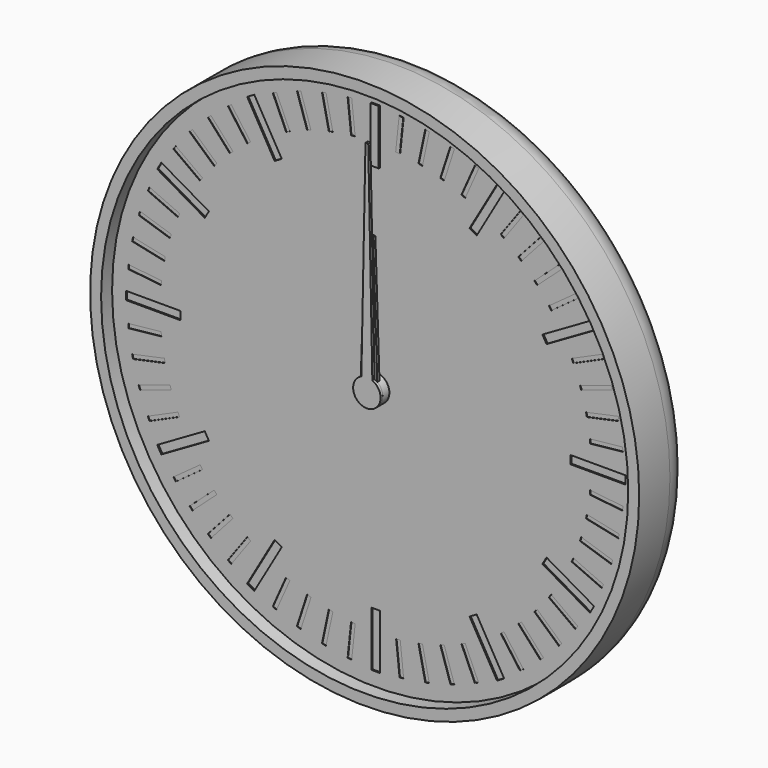
from build123d import *

# Parameters (mm, degrees)
F0_R      = 100
F1_DEPTH  = 24
F2_R      = 10
F3_T      = -4
F4_R      = 5
F4_R_2    = 3
F5_DEPTH  = 2
F6_DEPTH  = 19
F7_DEPTH  = 8
F9_DEPTH  = 4
F11_DEPTH = 4
F12_R     = 5
F12_R_2   = 3
F13_DEPTH = 2
F14_R     = 3
F15_DEPTH = 4
F17_DEPTH = 4
F18_R     = 3
F19_DEPTH = 2
F20_R     = 98
F20_R_2   = 5
F21_DEPTH = 1
F23_R     = 5
F23_R_2   = 3
F24_DEPTH = 2
F25_W     = 3
F25_H     = 20
F25_W_2   = 20
F25_H_2   = 3
F26_DEPTH = 0.5
F27_W     = 1.5
F27_H     = 12
F27_W_2   = 12
F27_H_2   = 1.5
F28_DEPTH = 0.2
F29_DEPTH = 1
F30_DEPTH = 0.4
F31_R     = 5
F31_R_2   = 3
F32_DEPTH = 5
F33_R     = 3
F34_DEPTH = 1
F36_DEPTH = 1


with BuildPart() as f1:
    # F0 (on Front) → F1 (new body)
    with BuildSketch(Plane.XZ):
        Circle(F0_R)
    extrude(amount=F1_DEPTH)

    # F2
    f2_edges = [f1.edges().sort_by_distance(p)[0] for p in [
        (-100, 0, 0),
    ]]
    fillet(f2_edges, radius=F2_R)

    # F3
    f3_openings = [f1.faces().sort_by_distance(p)[0] for p in [
        (0, -24, 0),
    ]]
    offset(amount=F3_T, openings=f3_openings)

    # F4 (on face) → F5 (join)
    with BuildSketch(Plane.XZ.offset(4)):
        Circle(F4_R)
        Circle(F4_R_2, mode=Mode.SUBTRACT)
        with Locations((40, 0)):
            Circle(F4_R)
        with Locations((40, 0)):
            Circle(F4_R_2, mode=Mode.SUBTRACT)
    extrude(amount=F5_DEPTH)


with BuildPart() as f6:
    # F6 (new): a face of the model
    f6_faces = [f1.part.faces().sort_by_distance(p)[0] for p in [
        (0, -4, 0),
    ]]
    extrude(f6_faces, amount=F6_DEPTH)

    # F8 (on face) → F9 (join)
    with BuildSketch(Plane.XZ.offset(6)):
        with BuildLine():
            ThreePointArc((9.2729637667, -1.3794085621), (9.3494561423, -0.6915886375), (9.375, 0))
            ThreePointArc((9.375, 0), (9.3494561423, 0.6915886375), (9.2729637667, 1.3794085621))
            ThreePointArc((9.2729637667, 1.3794085621), (8.9161548403, 2.8970343223), (8.3127812852, 4.3345463782))
            ThreePointArc((8.3127812852, 4.3345463782), (7.5845343223, 5.5104867402), (6.6911892658, 6.566476316))
            ThreePointArc((6.6911892658, 6.566476316), (5.5104867402, 7.5845343223), (4.1773988938, 8.3928519278))
            ThreePointArc((4.1773988938, 8.3928519278), (2.8970343223, 8.9161548403), (1.5536078905, 9.2453733036))
            ThreePointArc((1.5536078905, 9.2453733036), (0, 9.375), (-1.5536078905, 9.2453733036))
            ThreePointArc((-1.5536078905, 9.2453733036), (-2.8970343223, 8.9161548403), (-4.1773988938, 8.3928519278))
            ThreePointArc((-4.1773988938, 8.3928519278), (-5.5104867402, 7.5845343223), (-6.6911892658, 6.566476316))
            ThreePointArc((-6.6911892658, 6.566476316), (-7.5845343223, 5.5104867402), (-8.3127812852, 4.3345463782))
            ThreePointArc((-8.3127812852, 4.3345463782), (-8.9161548403, 2.8970343223), (-9.2729637667, 1.3794085621))
            ThreePointArc((-9.2729637667, 1.3794085621), (-9.375, 0), (-9.2729637667, -1.3794085621))
            ThreePointArc((-9.2729637667, -1.3794085621), (-8.9161548403, -2.8970343223), (-8.3127812852, -4.3345463782))
            ThreePointArc((-8.3127812852, -4.3345463782), (-7.5845343223, -5.5104867402), (-6.6911892658, -6.566476316))
            ThreePointArc((-6.6911892658, -6.566476316), (-5.5104867402, -7.5845343223), (-4.1773988938, -8.3928519278))
            ThreePointArc((-4.1773988938, -8.3928519278), (-2.8970343223, -8.9161548403), (-1.5536078905, -9.2453733036))
            ThreePointArc((-1.5536078905, -9.2453733036), (0, -9.375), (1.5536078905, -9.2453733036))
            ThreePointArc((1.5536078905, -9.2453733036), (2.8970343223, -8.9161548403), (4.1773988938, -8.3928519278))
            ThreePointArc((4.1773988938, -8.3928519278), (5.5104867402, -7.5845343223), (6.6911892658, -6.566476316))
            ThreePointArc((6.6911892658, -6.566476316), (7.5845343223, -5.5104867402), (8.3127812852, -4.3345463782))
            ThreePointArc((8.3127812852, -4.3345463782), (8.9161548403, -2.8970343223), (9.2729637667, -1.3794085621))
        make_face()
        with BuildLine():
            ThreePointArc((8.3127812852, 4.3345463782), (8.9161548403, 2.8970343223), (9.2729637667, 1.3794085621))
            Line((9.2729637667, 1.3794085621), (11.1823199426, 2.3946312492))
            Line((11.1823199426, 2.3946312492), (10.8182678729, 3.515068311))
            Line((10.8182678729, 3.515068311), (10.4542158031, 4.6355053728))
            Line((10.4542158031, 4.6355053728), (8.3127812852, 4.3345463782))
        make_face()
        with BuildLine():
            Line((11.1823199426, -2.3946312492), (9.2729637667, -1.3794085621))
            ThreePointArc((9.2729637667, -1.3794085621), (8.9161548403, -2.8970343223), (8.3127812852, -4.3345463782))
            Line((8.3127812852, -4.3345463782), (10.4542158031, -4.6355053728))
            Line((10.4542158031, -4.6355053728), (10.8182678729, -3.515068311))
            Line((10.8182678729, -3.515068311), (11.1823199426, -2.3946312492))
        make_face()
        with BuildLine():
            ThreePointArc((4.1773988938, 8.3928519278), (5.5104867402, 7.5845343223), (6.6911892658, 6.566476316))
            Line((6.6911892658, 6.566476316), (7.6391579371, 8.5101001246))
            Line((7.6391579371, 8.5101001246), (6.6860572448, 9.202568311))
            Line((6.6860572448, 9.202568311), (5.7329565525, 9.8950364974))
            Line((5.7329565525, 9.8950364974), (4.1773988938, 8.3928519278))
        make_face()
        with BuildLine():
            Line((7.6391579371, -8.5101001246), (6.6911892658, -6.566476316))
            ThreePointArc((6.6911892658, -6.566476316), (5.5104867402, -7.5845343223), (4.1773988938, -8.3928519278))
            Line((4.1773988938, -8.3928519278), (5.7329565525, -9.8950364974))
            Line((5.7329565525, -9.8950364974), (6.6860572448, -9.202568311))
            Line((6.6860572448, -9.202568311), (7.6391579371, -8.5101001246))
        make_face()
        with BuildLine():
            ThreePointArc((-1.5536078905, 9.2453733036), (0, 9.375), (1.5536078905, 9.2453733036))
            Line((1.5536078905, 9.2453733036), (1.1780972451, 11.375))
            Line((1.1780972451, 11.375), (0, 11.375))
            Line((0, 11.375), (-1.1780972451, 11.375))
            Line((-1.1780972451, 11.375), (-1.5536078905, 9.2453733036))
        make_face()
        with BuildLine():
            Line((1.1780972451, -11.375), (1.5536078905, -9.2453733036))
            ThreePointArc((1.5536078905, -9.2453733036), (0, -9.375), (-1.5536078905, -9.2453733036))
            Line((-1.5536078905, -9.2453733036), (-1.1780972451, -11.375))
            Line((-1.1780972451, -11.375), (0, -11.375))
            Line((0, -11.375), (1.1780972451, -11.375))
        make_face()
        with BuildLine():
            ThreePointArc((-6.6911892658, 6.566476316), (-5.5104867402, 7.5845343223), (-4.1773988938, 8.3928519278))
            Line((-4.1773988938, 8.3928519278), (-5.7329565525, 9.8950364974))
            Line((-5.7329565525, 9.8950364974), (-6.6860572448, 9.202568311))
            Line((-6.6860572448, 9.202568311), (-7.6391579371, 8.5101001246))
            Line((-7.6391579371, 8.5101001246), (-6.6911892658, 6.566476316))
        make_face()
        with BuildLine():
            Line((-5.7329565525, -9.8950364974), (-4.1773988938, -8.3928519278))
            ThreePointArc((-4.1773988938, -8.3928519278), (-5.5104867402, -7.5845343223), (-6.6911892658, -6.566476316))
            Line((-6.6911892658, -6.566476316), (-7.6391579371, -8.5101001246))
            Line((-7.6391579371, -8.5101001246), (-6.6860572448, -9.202568311))
            Line((-6.6860572448, -9.202568311), (-5.7329565525, -9.8950364974))
        make_face()
        with BuildLine():
            ThreePointArc((-9.2729637667, 1.3794085621), (-8.9161548403, 2.8970343223), (-8.3127812852, 4.3345463782))
            Line((-8.3127812852, 4.3345463782), (-10.4542158031, 4.6355053728))
            Line((-10.4542158031, 4.6355053728), (-10.8182678729, 3.515068311))
            Line((-10.8182678729, 3.515068311), (-11.1823199426, 2.3946312492))
            Line((-11.1823199426, 2.3946312492), (-9.2729637667, 1.3794085621))
        make_face()
        with BuildLine():
            Line((-10.4542158031, -4.6355053728), (-8.3127812852, -4.3345463782))
            ThreePointArc((-8.3127812852, -4.3345463782), (-8.9161548403, -2.8970343223), (-9.2729637667, -1.3794085621))
            Line((-9.2729637667, -1.3794085621), (-11.1823199426, -2.3946312492))
            Line((-11.1823199426, -2.3946312492), (-10.8182678729, -3.515068311))
            Line((-10.8182678729, -3.515068311), (-10.4542158031, -4.6355053728))
        make_face()
    extrude(amount=F9_DEPTH)

    # F35 (on face) → F36 (join)
    with BuildSketch(Plane.XZ.offset(23)):
        with BuildLine():
            ThreePointArc((-2, 4.582575695), (-2.7386127875, -4.1833001327), (5, 0))
            ThreePointArc((5, 0), (4.1833001327, 2.7386127875), (2, 4.582575695))
            ThreePointArc((2, 4.582575695), (0, 5), (-2, 4.582575695))
        make_face()
        with BuildLine():
            ThreePointArc((-2, 4.582575695), (0, 5), (2, 4.582575695))
            Line((2, 4.582575695), (0.5, 80))
            Line((0.5, 80), (0, 80))
            Line((0, 80), (-0.5, 80))
            Line((-0.5, 80), (-2, 4.582575695))
        make_face()
    extrude(amount=-F36_DEPTH)


with BuildPart() as f7:
    # F7 (new): a face of the model
    f7_faces = [f1.part.faces().sort_by_distance(p)[0] for p in [
        (40, -4, 0),
    ]]
    extrude(f7_faces, amount=F7_DEPTH)

    # F10 (on face) → F11 (join)
    with BuildSketch(Plane.XZ.offset(6)):
        with BuildLine():
            ThreePointArc((68.0833122289, -1.5307512065), (68.1145761255, -0.765659377), (68.125, 0))
            ThreePointArc((68.125, 0), (68.1145761255, 0.765659377), (68.0833122289, 1.5307512065))
            ThreePointArc((68.0833122289, 1.5307512065), (67.9709283072, 2.9398630294), (67.7878855489, 4.3415483093))
            ThreePointArc((67.7878855489, 4.3415483093), (67.5104012706, 5.8475163042), (67.1513634058, 7.3361495492))
            ThreePointArc((67.1513634058, 7.3361495492), (66.7484645208, 8.6911029668), (66.2779949294, 10.0241013309))
            ThreePointArc((66.2779949294, 10.0241013309), (65.6934659962, 11.4394680865), (65.0327697151, 12.8209229539))
            ThreePointArc((65.0327697151, 12.8209229539), (64.3569644814, 14.0625), (63.6196298356, 15.2685530234))
            ThreePointArc((63.6196298356, 15.2685530234), (62.7536029668, 16.5314602207), (61.8201238674, 17.7453605039))
            ThreePointArc((61.8201238674, 17.7453605039), (60.9009482166, 18.8192983038), (59.9289735785, 19.8456956821))
            ThreePointArc((59.9289735785, 19.8456956821), (58.8192983038, 20.9009482166), (57.6538339021, 21.8942406481))
            ThreePointArc((57.6538339021, 21.8942406481), (56.5314602207, 22.7536029668), (55.3673255461, 23.5554862093))
            ThreePointArc((55.3673255461, 23.5554862093), (54.0625, 24.3569644814), (52.7159866827, 25.0862374159))
            ThreePointArc((52.7159866827, 25.0862374159), (51.4394680865, 25.6934659962), (50.1340516468, 26.2357889574))
            ThreePointArc((50.1340516468, 26.2357889574), (48.6911029668, 26.7484645208), (47.2223898273, 27.1818452314))
            ThreePointArc((47.2223898273, 27.1818452314), (45.8475163042, 27.5104012706), (44.457871062, 27.7694618348))
            ThreePointArc((44.457871062, 27.7694618348), (42.9398630294, 27.9709283072), (41.4131398795, 28.0894759773))
            ThreePointArc((41.4131398795, 28.0894759773), (40, 28.125), (38.5868601205, 28.0894759773))
            ThreePointArc((38.5868601205, 28.0894759773), (37.0601369706, 27.9709283072), (35.542128938, 27.7694618348))
            ThreePointArc((35.542128938, 27.7694618348), (34.1524836958, 27.5104012706), (32.7776101727, 27.1818452314))
            ThreePointArc((32.7776101727, 27.1818452314), (31.3088970332, 26.7484645208), (29.8659483532, 26.2357889574))
            ThreePointArc((29.8659483532, 26.2357889574), (28.5605319135, 25.6934659962), (27.2840133173, 25.0862374159))
            ThreePointArc((27.2840133173, 25.0862374159), (25.9375, 24.3569644814), (24.6326744539, 23.5554862093))
            ThreePointArc((24.6326744539, 23.5554862093), (23.4685397793, 22.7536029668), (22.3461660979, 21.8942406481))
            ThreePointArc((22.3461660979, 21.8942406481), (21.1807016962, 20.9009482166), (20.0710264215, 19.8456956821))
            ThreePointArc((20.0710264215, 19.8456956821), (19.0990517834, 18.8192983038), (18.1798761326, 17.7453605039))
            ThreePointArc((18.1798761326, 17.7453605039), (17.2463970332, 16.5314602207), (16.3803701644, 15.2685530234))
            ThreePointArc((16.3803701644, 15.2685530234), (15.6430355186, 14.0625), (14.9672302849, 12.8209229539))
            ThreePointArc((14.9672302849, 12.8209229539), (14.3065340038, 11.4394680865), (13.7220050706, 10.0241013309))
            ThreePointArc((13.7220050706, 10.0241013309), (13.2515354792, 8.6911029668), (12.8486365942, 7.3361495492))
            ThreePointArc((12.8486365942, 7.3361495492), (12.4895987294, 5.8475163042), (12.2121144511, 4.3415483093))
            ThreePointArc((12.2121144511, 4.3415483093), (12.0290716928, 2.9398630294), (11.9166877711, 1.5307512065))
            ThreePointArc((11.9166877711, 1.5307512065), (11.875, 0), (11.9166877711, -1.5307512065))
            ThreePointArc((11.9166877711, -1.5307512065), (12.0290716928, -2.9398630294), (12.2121144511, -4.3415483093))
            ThreePointArc((12.2121144511, -4.3415483093), (12.4895987294, -5.8475163042), (12.8486365942, -7.3361495492))
            ThreePointArc((12.8486365942, -7.3361495492), (13.2515354792, -8.6911029668), (13.7220050706, -10.0241013309))
            ThreePointArc((13.7220050706, -10.0241013309), (14.3065340038, -11.4394680865), (14.9672302849, -12.8209229539))
            ThreePointArc((14.9672302849, -12.8209229539), (15.6430355186, -14.0625), (16.3803701644, -15.2685530234))
            ThreePointArc((16.3803701644, -15.2685530234), (17.2463970332, -16.5314602207), (18.1798761326, -17.7453605039))
            ThreePointArc((18.1798761326, -17.7453605039), (19.0990517834, -18.8192983038), (20.0710264215, -19.8456956821))
            ThreePointArc((20.0710264215, -19.8456956821), (21.1807016962, -20.9009482166), (22.3461660979, -21.8942406481))
            ThreePointArc((22.3461660979, -21.8942406481), (23.4685397793, -22.7536029668), (24.6326744539, -23.5554862093))
            ThreePointArc((24.6326744539, -23.5554862093), (25.9375, -24.3569644814), (27.2840133173, -25.0862374159))
            ThreePointArc((27.2840133173, -25.0862374159), (28.5605319135, -25.6934659962), (29.8659483532, -26.2357889574))
            ThreePointArc((29.8659483532, -26.2357889574), (31.3088970332, -26.7484645208), (32.7776101727, -27.1818452314))
            ThreePointArc((32.7776101727, -27.1818452314), (34.1524836958, -27.5104012706), (35.542128938, -27.7694618348))
            ThreePointArc((35.542128938, -27.7694618348), (37.0601369706, -27.9709283072), (38.5868601205, -28.0894759773))
            ThreePointArc((38.5868601205, -28.0894759773), (40, -28.125), (41.4131398795, -28.0894759773))
            ThreePointArc((41.4131398795, -28.0894759773), (42.9398630294, -27.9709283072), (44.457871062, -27.7694618348))
            ThreePointArc((44.457871062, -27.7694618348), (45.8475163042, -27.5104012706), (47.2223898273, -27.1818452314))
            ThreePointArc((47.2223898273, -27.1818452314), (48.6911029668, -26.7484645208), (50.1340516468, -26.2357889574))
            ThreePointArc((50.1340516468, -26.2357889574), (51.4394680865, -25.6934659962), (52.7159866827, -25.0862374159))
            ThreePointArc((52.7159866827, -25.0862374159), (54.0625, -24.3569644814), (55.3673255461, -23.5554862093))
            ThreePointArc((55.3673255461, -23.5554862093), (56.5314602207, -22.7536029668), (57.6538339021, -21.8942406481))
            ThreePointArc((57.6538339021, -21.8942406481), (58.8192983038, -20.9009482166), (59.9289735785, -19.8456956821))
            ThreePointArc((59.9289735785, -19.8456956821), (60.9009482166, -18.8192983038), (61.8201238674, -17.7453605039))
            ThreePointArc((61.8201238674, -17.7453605039), (62.7536029668, -16.5314602207), (63.6196298356, -15.2685530234))
            ThreePointArc((63.6196298356, -15.2685530234), (64.3569644814, -14.0625), (65.0327697151, -12.8209229539))
            ThreePointArc((65.0327697151, -12.8209229539), (65.6934659962, -11.4394680865), (66.2779949294, -10.0241013309))
            ThreePointArc((66.2779949294, -10.0241013309), (66.7484645208, -8.6911029668), (67.1513634058, -7.3361495492))
            ThreePointArc((67.1513634058, -7.3361495492), (67.5104012706, -5.8475163042), (67.7878855489, -4.3415483093))
            ThreePointArc((67.7878855489, -4.3415483093), (67.9709283072, -2.9398630294), (68.0833122289, -1.5307512065))
        make_face()
        with BuildLine():
            ThreePointArc((68.0833122289, 1.5307512065), (68.1145761255, 0.765659377), (68.125, 0))
            ThreePointArc((68.125, 0), (68.1145761255, -0.765659377), (68.0833122289, -1.5307512065))
            Line((68.0833122289, -1.5307512065), (70.0833122289, -1.1780972451))
            Line((70.0833122289, -1.1780972451), (70.0833122289, 0))
            Line((70.0833122289, 0), (70.0833122289, 1.1780972451))
            Line((70.0833122289, 1.1780972451), (68.0833122289, 1.5307512065))
        make_face()
        with BuildLine():
            ThreePointArc((67.1513634058, 7.3361495492), (67.5104012706, 5.8475163042), (67.7878855489, 4.3415483093))
            Line((67.7878855489, 4.3415483093), (69.670859869, 5.1023193172))
            Line((69.670859869, 5.1023193172), (69.4259196788, 6.2546723109))
            Line((69.4259196788, 6.2546723109), (69.1809794886, 7.4070253046))
            Line((69.1809794886, 7.4070253046), (67.1513634058, 7.3361495492))
        make_face()
        with BuildLine():
            Line((69.670859869, -5.1023193172), (67.7878855489, -4.3415483093))
            ThreePointArc((67.7878855489, -4.3415483093), (67.5104012706, -5.8475163042), (67.1513634058, -7.3361495492))
            Line((67.1513634058, -7.3361495492), (69.1809794886, -7.4070253046))
            Line((69.1809794886, -7.4070253046), (69.4259196788, -6.2546723109))
            Line((69.4259196788, -6.2546723109), (69.670859869, -5.1023193172))
        make_face()
        with BuildLine():
            ThreePointArc((65.0327697151, 12.8209229539), (65.6934659962, 11.4394680865), (66.2779949294, 10.0241013309))
            Line((66.2779949294, 10.0241013309), (67.9616485562, 11.1597400416))
            Line((67.9616485562, 11.1597400416), (67.4824732375, 12.2359854286))
            Line((67.4824732375, 12.2359854286), (67.0032979188, 13.3122308155))
            Line((67.0032979188, 13.3122308155), (65.0327697151, 12.8209229539))
        make_face()
        with BuildLine():
            Line((67.9616485562, -11.1597400416), (66.2779949294, -10.0241013309))
            ThreePointArc((66.2779949294, -10.0241013309), (65.6934659962, -11.4394680865), (65.0327697151, -12.8209229539))
            Line((65.0327697151, -12.8209229539), (67.0032979188, -13.3122308155))
            Line((67.0032979188, -13.3122308155), (67.4824732375, -12.2359854286))
            Line((67.4824732375, -12.2359854286), (67.9616485562, -11.1597400416))
        make_face()
        with BuildLine():
            ThreePointArc((61.8201238674, 17.7453605039), (62.7536029668, 16.5314602207), (63.6196298356, 15.2685530234))
            Line((63.6196298356, 15.2685530234), (65.0303790267, 16.7294265759))
            Line((65.0303790267, 16.7294265759), (64.3379108402, 17.6825272682))
            Line((64.3379108402, 17.6825272682), (63.6454426538, 18.6356279605))
            Line((63.6454426538, 18.6356279605), (61.8201238674, 17.7453605039))
        make_face()
        with BuildLine():
            Line((65.0303790267, -16.7294265759), (63.6196298356, -15.2685530234))
            ThreePointArc((63.6196298356, -15.2685530234), (62.7536029668, -16.5314602207), (61.8201238674, -17.7453605039))
            Line((61.8201238674, -17.7453605039), (63.6454426538, -18.6356279605))
            Line((63.6454426538, -18.6356279605), (64.3379108402, -17.6825272682))
            Line((64.3379108402, -17.6825272682), (65.0303790267, -16.7294265759))
        make_face()
        with BuildLine():
            ThreePointArc((57.6538339021, 21.8942406481), (58.8192983038, 20.9009482166), (59.9289735785, 19.8456956821))
            Line((59.9289735785, 19.8456956821), (61.0051618246, 21.5679568921))
            Line((61.0051618246, 21.5679568921), (60.129664953, 22.3562578161))
            Line((60.129664953, 22.3562578161), (59.2541680814, 23.1445587401))
            Line((59.2541680814, 23.1445587401), (57.6538339021, 21.8942406481))
        make_face()
        with BuildLine():
            Line((61.0051618246, -21.5679568921), (59.9289735785, -19.8456956821))
            ThreePointArc((59.9289735785, -19.8456956821), (58.8192983038, -20.9009482166), (57.6538339021, -21.8942406481))
            Line((57.6538339021, -21.8942406481), (59.2541680814, -23.1445587401))
            Line((59.2541680814, -23.1445587401), (60.129664953, -22.3562578161))
            Line((60.129664953, -22.3562578161), (61.0051618246, -21.5679568921))
        make_face()
        with BuildLine():
            ThreePointArc((52.7159866827, 25.0862374159), (54.0625, 24.3569644814), (55.3673255461, 23.5554862093))
            Line((55.3673255461, 23.5554862093), (56.0619182568, 25.4638639976))
            Line((56.0619182568, 25.4638639976), (55.0416561144, 26.0529126202))
            Line((55.0416561144, 26.0529126202), (54.021393972, 26.6419612427))
            Line((54.021393972, 26.6419612427), (52.7159866827, 25.0862374159))
        make_face()
        with BuildLine():
            Line((56.0619182568, -25.4638639976), (55.3673255461, -23.5554862093))
            ThreePointArc((55.3673255461, -23.5554862093), (54.0625, -24.3569644814), (52.7159866827, -25.0862374159))
            Line((52.7159866827, -25.0862374159), (54.021393972, -26.6419612427))
            Line((54.021393972, -26.6419612427), (55.0416561144, -26.0529126202))
            Line((55.0416561144, -26.0529126202), (56.0619182568, -25.4638639976))
        make_face()
        with BuildLine():
            ThreePointArc((47.2223898273, 27.1818452314), (48.6911029668, 26.7484645208), (50.1340516468, 26.2357889574))
            Line((50.1340516468, 26.2357889574), (50.4166917876, 28.2468780572))
            Line((50.4166917876, 28.2468780572), (49.2962547258, 28.610930127))
            Line((49.2962547258, 28.610930127), (48.175817664, 28.9749821968))
            Line((48.175817664, 28.9749821968), (47.2223898273, 27.1818452314))
        make_face()
        with BuildLine():
            Line((50.4166917876, -28.2468780572), (50.1340516468, -26.2357889574))
            ThreePointArc((50.1340516468, -26.2357889574), (48.6911029668, -26.7484645208), (47.2223898273, -27.1818452314))
            Line((47.2223898273, -27.1818452314), (48.175817664, -28.9749821968))
            Line((48.175817664, -28.9749821968), (49.2962547258, -28.610930127))
            Line((49.2962547258, -28.610930127), (50.4166917876, -28.2468780572))
        make_face()
        with BuildLine():
            ThreePointArc((41.4131398795, 28.0894759773), (42.9398630294, 27.9709283072), (44.457871062, 27.7694618348))
            Line((44.457871062, 27.7694618348), (44.3162059024, 29.7953680022))
            Line((44.3162059024, 29.7953680022), (43.1445623973, 29.9185126968))
            Line((43.1445623973, 29.9185126968), (41.9729188922, 30.0416573914))
            Line((41.9729188922, 30.0416573914), (41.4131398795, 28.0894759773))
        make_face()
        with BuildLine():
            Line((44.3162059024, -29.7953680022), (44.457871062, -27.7694618348))
            ThreePointArc((44.457871062, -27.7694618348), (42.9398630294, -27.9709283072), (41.4131398795, -28.0894759773))
            Line((41.4131398795, -28.0894759773), (41.9729188922, -30.0416573914))
            Line((41.9729188922, -30.0416573914), (43.1445623973, -29.9185126968))
            Line((43.1445623973, -29.9185126968), (44.3162059024, -29.7953680022))
        make_face()
        with BuildLine():
            ThreePointArc((35.542128938, 27.7694618348), (37.0601369706, 27.9709283072), (38.5868601205, 28.0894759773))
            Line((38.5868601205, 28.0894759773), (38.0270811078, 30.0416573914))
            Line((38.0270811078, 30.0416573914), (36.8554376027, 29.9185126968))
            Line((36.8554376027, 29.9185126968), (35.6837940976, 29.7953680022))
            Line((35.6837940976, 29.7953680022), (35.542128938, 27.7694618348))
        make_face()
        with BuildLine():
            Line((38.0270811078, -30.0416573914), (38.5868601205, -28.0894759773))
            ThreePointArc((38.5868601205, -28.0894759773), (37.0601369706, -27.9709283072), (35.542128938, -27.7694618348))
            Line((35.542128938, -27.7694618348), (35.6837940976, -29.7953680022))
            Line((35.6837940976, -29.7953680022), (36.8554376027, -29.9185126968))
            Line((36.8554376027, -29.9185126968), (38.0270811078, -30.0416573914))
        make_face()
        with BuildLine():
            ThreePointArc((29.8659483532, 26.2357889574), (31.3088970332, 26.7484645208), (32.7776101727, 27.1818452314))
            Line((32.7776101727, 27.1818452314), (31.824182336, 28.9749821968))
            Line((31.824182336, 28.9749821968), (30.7037452742, 28.610930127))
            Line((30.7037452742, 28.610930127), (29.5833082124, 28.2468780572))
            Line((29.5833082124, 28.2468780572), (29.8659483532, 26.2357889574))
        make_face()
        with BuildLine():
            Line((31.824182336, -28.9749821968), (32.7776101727, -27.1818452314))
            ThreePointArc((32.7776101727, -27.1818452314), (31.3088970332, -26.7484645208), (29.8659483532, -26.2357889574))
            Line((29.8659483532, -26.2357889574), (29.5833082124, -28.2468780572))
            Line((29.5833082124, -28.2468780572), (30.7037452742, -28.610930127))
            Line((30.7037452742, -28.610930127), (31.824182336, -28.9749821968))
        make_face()
        with BuildLine():
            ThreePointArc((24.6326744539, 23.5554862093), (25.9375, 24.3569644814), (27.2840133173, 25.0862374159))
            Line((27.2840133173, 25.0862374159), (25.978606028, 26.6419612427))
            Line((25.978606028, 26.6419612427), (24.9583438856, 26.0529126202))
            Line((24.9583438856, 26.0529126202), (23.9380817432, 25.4638639976))
            Line((23.9380817432, 25.4638639976), (24.6326744539, 23.5554862093))
        make_face()
        with BuildLine():
            Line((25.978606028, -26.6419612427), (27.2840133173, -25.0862374159))
            ThreePointArc((27.2840133173, -25.0862374159), (25.9375, -24.3569644814), (24.6326744539, -23.5554862093))
            Line((24.6326744539, -23.5554862093), (23.9380817432, -25.4638639976))
            Line((23.9380817432, -25.4638639976), (24.9583438856, -26.0529126202))
            Line((24.9583438856, -26.0529126202), (25.978606028, -26.6419612427))
        make_face()
        with BuildLine():
            ThreePointArc((20.0710264215, 19.8456956821), (21.1807016962, 20.9009482166), (22.3461660979, 21.8942406481))
            Line((22.3461660979, 21.8942406481), (20.7458319186, 23.1445587401))
            Line((20.7458319186, 23.1445587401), (19.870335047, 22.3562578161))
            Line((19.870335047, 22.3562578161), (18.9948381754, 21.5679568921))
            Line((18.9948381754, 21.5679568921), (20.0710264215, 19.8456956821))
        make_face()
        with BuildLine():
            Line((20.7458319186, -23.1445587401), (22.3461660979, -21.8942406481))
            ThreePointArc((22.3461660979, -21.8942406481), (21.1807016962, -20.9009482166), (20.0710264215, -19.8456956821))
            Line((20.0710264215, -19.8456956821), (18.9948381754, -21.5679568921))
            Line((18.9948381754, -21.5679568921), (19.870335047, -22.3562578161))
            Line((19.870335047, -22.3562578161), (20.7458319186, -23.1445587401))
        make_face()
        with BuildLine():
            ThreePointArc((16.3803701644, 15.2685530234), (17.2463970332, 16.5314602207), (18.1798761326, 17.7453605039))
            Line((18.1798761326, 17.7453605039), (16.3545573462, 18.6356279605))
            Line((16.3545573462, 18.6356279605), (15.6620891598, 17.6825272682))
            Line((15.6620891598, 17.6825272682), (14.9696209733, 16.7294265759))
            Line((14.9696209733, 16.7294265759), (16.3803701644, 15.2685530234))
        make_face()
        with BuildLine():
            Line((16.3545573462, -18.6356279605), (18.1798761326, -17.7453605039))
            ThreePointArc((18.1798761326, -17.7453605039), (17.2463970332, -16.5314602207), (16.3803701644, -15.2685530234))
            Line((16.3803701644, -15.2685530234), (14.9696209733, -16.7294265759))
            Line((14.9696209733, -16.7294265759), (15.6620891598, -17.6825272682))
            Line((15.6620891598, -17.6825272682), (16.3545573462, -18.6356279605))
        make_face()
        with BuildLine():
            ThreePointArc((13.7220050706, 10.0241013309), (14.3065340038, 11.4394680865), (14.9672302849, 12.8209229539))
            Line((14.9672302849, 12.8209229539), (12.9967020812, 13.3122308155))
            Line((12.9967020812, 13.3122308155), (12.5175267625, 12.2359854286))
            Line((12.5175267625, 12.2359854286), (12.0383514438, 11.1597400416))
            Line((12.0383514438, 11.1597400416), (13.7220050706, 10.0241013309))
        make_face()
        with BuildLine():
            Line((12.9967020812, -13.3122308155), (14.9672302849, -12.8209229539))
            ThreePointArc((14.9672302849, -12.8209229539), (14.3065340038, -11.4394680865), (13.7220050706, -10.0241013309))
            Line((13.7220050706, -10.0241013309), (12.0383514438, -11.1597400416))
            Line((12.0383514438, -11.1597400416), (12.5175267625, -12.2359854286))
            Line((12.5175267625, -12.2359854286), (12.9967020812, -13.3122308155))
        make_face()
        with BuildLine():
            ThreePointArc((12.2121144511, 4.3415483093), (12.4895987294, 5.8475163042), (12.8486365942, 7.3361495492))
            Line((12.8486365942, 7.3361495492), (10.8190205114, 7.4070253046))
            Line((10.8190205114, 7.4070253046), (10.5740803212, 6.2546723109))
            Line((10.5740803212, 6.2546723109), (10.329140131, 5.1023193172))
            Line((10.329140131, 5.1023193172), (12.2121144511, 4.3415483093))
        make_face()
        with BuildLine():
            Line((10.8190205114, -7.4070253046), (12.8486365942, -7.3361495492))
            ThreePointArc((12.8486365942, -7.3361495492), (12.4895987294, -5.8475163042), (12.2121144511, -4.3415483093))
            Line((12.2121144511, -4.3415483093), (10.329140131, -5.1023193172))
            Line((10.329140131, -5.1023193172), (10.5740803212, -6.2546723109))
            Line((10.5740803212, -6.2546723109), (10.8190205114, -7.4070253046))
        make_face()
        with BuildLine():
            ThreePointArc((11.9166877711, -1.5307512065), (11.875, 0), (11.9166877711, 1.5307512065))
            Line((11.9166877711, 1.5307512065), (9.9166877711, 1.1780972451))
            Line((9.9166877711, 1.1780972451), (9.9166877711, 0))
            Line((9.9166877711, 0), (9.9166877711, -1.1780972451))
            Line((9.9166877711, -1.1780972451), (11.9166877711, -1.5307512065))
        make_face()
    extrude(amount=F11_DEPTH)

    # F16 (on face) → F17 (join)
    with BuildSketch(Plane.XZ.offset(12)):
        with BuildLine():
            ThreePointArc((47.4288750323, -1.0304444454), (47.4821976298, -0.5164480894), (47.5, 0))
            ThreePointArc((47.5, 0), (47.4821976298, 0.5164480894), (47.4288750323, 1.0304444454))
            ThreePointArc((47.4288750323, 1.0304444454), (47.1329238722, 2.3176274578), (46.6157661985, 3.532936117))
            ThreePointArc((46.6157661985, 3.532936117), (46.0676274578, 4.4083893922), (45.4044061018, 5.2002302532))
            ThreePointArc((45.4044061018, 5.2002302532), (44.4083893922, 6.0676274578), (43.2756595386, 6.7468551628))
            ThreePointArc((43.2756595386, 6.7468551628), (42.3176274578, 7.1329238722), (41.3156377295, 7.3837048536))
            ThreePointArc((41.3156377295, 7.3837048536), (40, 7.5), (38.6843622705, 7.3837048536))
            ThreePointArc((38.6843622705, 7.3837048536), (37.6823725422, 7.1329238722), (36.7243404614, 6.7468551628))
            ThreePointArc((36.7243404614, 6.7468551628), (35.5916106078, 6.0676274578), (34.5955938982, 5.2002302532))
            ThreePointArc((34.5955938982, 5.2002302532), (33.9323725422, 4.4083893922), (33.3842338015, 3.532936117))
            ThreePointArc((33.3842338015, 3.532936117), (32.8670761278, 2.3176274578), (32.5711249677, 1.0304444454))
            ThreePointArc((32.5711249677, 1.0304444454), (32.5, 0), (32.5711249677, -1.0304444454))
            ThreePointArc((32.5711249677, -1.0304444454), (32.8670761278, -2.3176274578), (33.3842338015, -3.532936117))
            ThreePointArc((33.3842338015, -3.532936117), (33.9323725422, -4.4083893922), (34.5955938982, -5.2002302532))
            ThreePointArc((34.5955938982, -5.2002302532), (35.5916106078, -6.0676274578), (36.7243404614, -6.7468551628))
            ThreePointArc((36.7243404614, -6.7468551628), (37.6823725422, -7.1329238722), (38.6843622705, -7.3837048536))
            ThreePointArc((38.6843622705, -7.3837048536), (40, -7.5), (41.3156377295, -7.3837048536))
            ThreePointArc((41.3156377295, -7.3837048536), (42.3176274578, -7.1329238722), (43.2756595386, -6.7468551628))
            ThreePointArc((43.2756595386, -6.7468551628), (44.4083893922, -6.0676274578), (45.4044061018, -5.2002302532))
            ThreePointArc((45.4044061018, -5.2002302532), (46.0676274578, -4.4083893922), (46.6157661985, -3.532936117))
            ThreePointArc((46.6157661985, -3.532936117), (47.1329238722, -2.3176274578), (47.4288750323, -1.0304444454))
        make_face()
        with BuildLine():
            ThreePointArc((46.6157661985, 3.532936117), (47.1329238722, 2.3176274578), (47.4288750323, 1.0304444454))
            Line((47.4288750323, 1.0304444454), (49.3262785606, 2.0393117971))
            Line((49.3262785606, 2.0393117971), (48.743795249, 3.832011096))
            Line((48.743795249, 3.832011096), (46.6157661985, 3.532936117))
        make_face()
        with BuildLine():
            Line((49.3262785606, -2.0393117971), (47.4288750323, -1.0304444454))
            ThreePointArc((47.4288750323, -1.0304444454), (47.1329238722, -2.3176274578), (46.6157661985, -3.532936117))
            Line((46.6157661985, -3.532936117), (48.743795249, -3.832011096))
            Line((48.743795249, -3.832011096), (49.3262785606, -2.0393117971))
        make_face()
        with BuildLine():
            ThreePointArc((43.2756595386, 6.7468551628), (44.4083893922, 6.0676274578), (45.4044061018, 5.2002302532))
            Line((45.4044061018, 5.2002302532), (46.3464404506, 7.1316868974))
            Line((46.3464404506, 7.1316868974), (44.8214793429, 8.2396359957))
            Line((44.8214793429, 8.2396359957), (43.2756595386, 6.7468551628))
        make_face()
        with BuildLine():
            Line((46.3464404506, -7.1316868974), (45.4044061018, -5.2002302532))
            ThreePointArc((45.4044061018, -5.2002302532), (44.4083893922, -6.0676274578), (43.2756595386, -6.7468551628))
            Line((43.2756595386, -6.7468551628), (44.8214793429, -8.2396359957))
            Line((44.8214793429, -8.2396359957), (46.3464404506, -7.1316868974))
        make_face()
        with BuildLine():
            ThreePointArc((38.6843622705, 7.3837048536), (40, 7.5), (41.3156377295, 7.3837048536))
            Line((41.3156377295, 7.3837048536), (40.9424777961, 9.5))
            Line((40.9424777961, 9.5), (39.0575222039, 9.5))
            Line((39.0575222039, 9.5), (38.6843622705, 7.3837048536))
        make_face()
        with BuildLine():
            Line((40.9424777961, -9.5), (41.3156377295, -7.3837048536))
            ThreePointArc((41.3156377295, -7.3837048536), (40, -7.5), (38.6843622705, -7.3837048536))
            Line((38.6843622705, -7.3837048536), (39.0575222039, -9.5))
            Line((39.0575222039, -9.5), (40.9424777961, -9.5))
        make_face()
        with BuildLine():
            ThreePointArc((34.5955938982, 5.2002302532), (35.5916106078, 6.0676274578), (36.7243404614, 6.7468551628))
            Line((36.7243404614, 6.7468551628), (35.1785206571, 8.2396359957))
            Line((35.1785206571, 8.2396359957), (33.6535595494, 7.1316868974))
            Line((33.6535595494, 7.1316868974), (34.5955938982, 5.2002302532))
        make_face()
        with BuildLine():
            Line((35.1785206571, -8.2396359957), (36.7243404614, -6.7468551628))
            ThreePointArc((36.7243404614, -6.7468551628), (35.5916106078, -6.0676274578), (34.5955938982, -5.2002302532))
            Line((34.5955938982, -5.2002302532), (33.6535595494, -7.1316868974))
            Line((33.6535595494, -7.1316868974), (35.1785206571, -8.2396359957))
        make_face()
        with BuildLine():
            ThreePointArc((32.5711249677, 1.0304444454), (32.8670761278, 2.3176274578), (33.3842338015, 3.532936117))
            Line((33.3842338015, 3.532936117), (31.256204751, 3.832011096))
            Line((31.256204751, 3.832011096), (30.6737214394, 2.0393117971))
            Line((30.6737214394, 2.0393117971), (32.5711249677, 1.0304444454))
        make_face()
        with BuildLine():
            Line((31.256204751, -3.832011096), (33.3842338015, -3.532936117))
            ThreePointArc((33.3842338015, -3.532936117), (32.8670761278, -2.3176274578), (32.5711249677, -1.0304444454))
            Line((32.5711249677, -1.0304444454), (30.6737214394, -2.0393117971))
            Line((30.6737214394, -2.0393117971), (31.256204751, -3.832011096))
        make_face()
    extrude(amount=F17_DEPTH)

    # F18 (on face) → F19 (join)
    with BuildSketch(Plane.XZ.offset(16)):
        with Locations((40, 0)):
            Circle(F18_R)
    extrude(amount=F19_DEPTH)


with BuildPart() as f13:
    # F12 (on face) → F13 (new body)
    with BuildSketch(Plane.XZ.offset(10)):
        Circle(F12_R)
        Circle(F12_R_2, mode=Mode.SUBTRACT)
    extrude(amount=F13_DEPTH)

    # F14 (on face) → F15 (join)
    with BuildSketch(Plane.XZ.offset(12)):
        with BuildLine():
            ThreePointArc((29.9718156995, -1.3001014101), (29.9929530972, -0.6502034357), (30, 0))
            ThreePointArc((30, 0), (29.9929530972, 0.6502034357), (29.9718156995, 1.3001014101))
            ThreePointArc((29.9718156995, 1.3001014101), (29.907520012, 2.3537728718), (29.8061935814, 3.4045299509))
            ThreePointArc((29.8061935814, 3.4045299509), (29.6306502179, 4.6930339512), (29.3994322443, 5.9727199596))
            ThreePointArc((29.3994322443, 5.9727199596), (29.1710976119, 7.0033609157), (28.9066440563, 8.0253304855))
            ThreePointArc((28.9066440563, 8.0253304855), (28.5316954889, 9.2705098312), (28.1031371961, 10.4982703213))
            ThreePointArc((28.1031371961, 10.4982703213), (27.7163859753, 11.480502971), (27.2953170189, 12.448520749))
            ThreePointArc((27.2953170189, 12.448520749), (26.7301957257, 13.6197149922), (26.1148496411, 14.765318426))
            ThreePointArc((26.1148496411, 14.765318426), (25.5792049306, 15.6749569415), (25.0118886885, 16.5651871174))
            ThreePointArc((25.0118886885, 16.5651871174), (24.2705098312, 17.6335575688), (23.4835278178, 18.6687953878))
            ThreePointArc((23.4835278178, 18.6687953878), (22.812178968, 19.4834414499), (22.1125846489, 20.2739636023))
            ThreePointArc((22.1125846489, 20.2739636023), (21.2132034356, 21.2132034356), (20.2739636023, 22.1125846489))
            ThreePointArc((20.2739636023, 22.1125846489), (19.4834414499, 22.812178968), (18.6687953878, 23.4835278178))
            ThreePointArc((18.6687953878, 23.4835278178), (17.6335575688, 24.2705098312), (16.5651871174, 25.0118886885))
            ThreePointArc((16.5651871174, 25.0118886885), (15.6749569415, 25.5792049306), (14.765318426, 26.1148496411))
            ThreePointArc((14.765318426, 26.1148496411), (13.6197149922, 26.7301957257), (12.448520749, 27.2953170189))
            ThreePointArc((12.448520749, 27.2953170189), (11.480502971, 27.7163859753), (10.4982703213, 28.1031371961))
            ThreePointArc((10.4982703213, 28.1031371961), (9.2705098312, 28.5316954889), (8.0253304855, 28.9066440563))
            ThreePointArc((8.0253304855, 28.9066440563), (7.0033609157, 29.1710976119), (5.9727199596, 29.3994322443))
            ThreePointArc((5.9727199596, 29.3994322443), (4.6930339512, 29.6306502179), (3.4045299509, 29.8061935814))
            ThreePointArc((3.4045299509, 29.8061935814), (2.3537728718, 29.907520012), (1.3001014101, 29.9718156995))
            ThreePointArc((1.3001014101, 29.9718156995), (0, 30), (-1.3001014101, 29.9718156995))
            ThreePointArc((-1.3001014101, 29.9718156995), (-2.3537728718, 29.907520012), (-3.4045299509, 29.8061935814))
            ThreePointArc((-3.4045299509, 29.8061935814), (-4.6930339512, 29.6306502179), (-5.9727199596, 29.3994322443))
            ThreePointArc((-5.9727199596, 29.3994322443), (-7.0033609157, 29.1710976119), (-8.0253304855, 28.9066440563))
            ThreePointArc((-8.0253304855, 28.9066440563), (-9.2705098312, 28.5316954889), (-10.4982703213, 28.1031371961))
            ThreePointArc((-10.4982703213, 28.1031371961), (-11.480502971, 27.7163859753), (-12.448520749, 27.2953170189))
            ThreePointArc((-12.448520749, 27.2953170189), (-13.6197149922, 26.7301957257), (-14.765318426, 26.1148496411))
            ThreePointArc((-14.765318426, 26.1148496411), (-15.6749569415, 25.5792049306), (-16.5651871174, 25.0118886885))
            ThreePointArc((-16.5651871174, 25.0118886885), (-17.6335575688, 24.2705098312), (-18.6687953878, 23.4835278178))
            ThreePointArc((-18.6687953878, 23.4835278178), (-19.4834414499, 22.812178968), (-20.2739636023, 22.1125846489))
            ThreePointArc((-20.2739636023, 22.1125846489), (-21.2132034356, 21.2132034356), (-22.1125846489, 20.2739636023))
            ThreePointArc((-22.1125846489, 20.2739636023), (-22.812178968, 19.4834414499), (-23.4835278178, 18.6687953878))
            ThreePointArc((-23.4835278178, 18.6687953878), (-24.2705098312, 17.6335575688), (-25.0118886885, 16.5651871174))
            ThreePointArc((-25.0118886885, 16.5651871174), (-25.5792049306, 15.6749569415), (-26.1148496411, 14.765318426))
            ThreePointArc((-26.1148496411, 14.765318426), (-26.7301957257, 13.6197149922), (-27.2953170189, 12.448520749))
            ThreePointArc((-27.2953170189, 12.448520749), (-27.7163859753, 11.480502971), (-28.1031371961, 10.4982703213))
            ThreePointArc((-28.1031371961, 10.4982703213), (-28.5316954889, 9.2705098312), (-28.9066440563, 8.0253304855))
            ThreePointArc((-28.9066440563, 8.0253304855), (-29.1710976119, 7.0033609157), (-29.3994322443, 5.9727199596))
            ThreePointArc((-29.3994322443, 5.9727199596), (-29.6306502179, 4.6930339512), (-29.8061935814, 3.4045299509))
            ThreePointArc((-29.8061935814, 3.4045299509), (-29.907520012, 2.3537728718), (-29.9718156995, 1.3001014101))
            ThreePointArc((-29.9718156995, 1.3001014101), (-30, 0), (-29.9718156995, -1.3001014101))
            ThreePointArc((-29.9718156995, -1.3001014101), (-29.907520012, -2.3537728718), (-29.8061935814, -3.4045299509))
            ThreePointArc((-29.8061935814, -3.4045299509), (-29.6306502179, -4.6930339512), (-29.3994322443, -5.9727199596))
            ThreePointArc((-29.3994322443, -5.9727199596), (-29.1710976119, -7.0033609157), (-28.9066440563, -8.0253304855))
            ThreePointArc((-28.9066440563, -8.0253304855), (-28.5316954889, -9.2705098312), (-28.1031371961, -10.4982703213))
            ThreePointArc((-28.1031371961, -10.4982703213), (-27.7163859753, -11.480502971), (-27.2953170189, -12.448520749))
            ThreePointArc((-27.2953170189, -12.448520749), (-26.7301957257, -13.6197149922), (-26.1148496411, -14.765318426))
            ThreePointArc((-26.1148496411, -14.765318426), (-25.5792049306, -15.6749569415), (-25.0118886885, -16.5651871174))
            ThreePointArc((-25.0118886885, -16.5651871174), (-24.2705098312, -17.6335575688), (-23.4835278178, -18.6687953878))
            ThreePointArc((-23.4835278178, -18.6687953878), (-22.812178968, -19.4834414499), (-22.1125846489, -20.2739636023))
            ThreePointArc((-22.1125846489, -20.2739636023), (-21.2132034356, -21.2132034356), (-20.2739636023, -22.1125846489))
            ThreePointArc((-20.2739636023, -22.1125846489), (-19.4834414499, -22.812178968), (-18.6687953878, -23.4835278178))
            ThreePointArc((-18.6687953878, -23.4835278178), (-17.6335575688, -24.2705098312), (-16.5651871174, -25.0118886885))
            ThreePointArc((-16.5651871174, -25.0118886885), (-15.6749569415, -25.5792049306), (-14.765318426, -26.1148496411))
            ThreePointArc((-14.765318426, -26.1148496411), (-13.6197149922, -26.7301957257), (-12.448520749, -27.2953170189))
            ThreePointArc((-12.448520749, -27.2953170189), (-11.480502971, -27.7163859753), (-10.4982703213, -28.1031371961))
            ThreePointArc((-10.4982703213, -28.1031371961), (-9.2705098312, -28.5316954889), (-8.0253304855, -28.9066440563))
            ThreePointArc((-8.0253304855, -28.9066440563), (-7.0033609157, -29.1710976119), (-5.9727199596, -29.3994322443))
            ThreePointArc((-5.9727199596, -29.3994322443), (-4.6930339512, -29.6306502179), (-3.4045299509, -29.8061935814))
            ThreePointArc((-3.4045299509, -29.8061935814), (-2.3537728718, -29.907520012), (-1.3001014101, -29.9718156995))
            ThreePointArc((-1.3001014101, -29.9718156995), (0, -30), (1.3001014101, -29.9718156995))
            ThreePointArc((1.3001014101, -29.9718156995), (2.3537728718, -29.907520012), (3.4045299509, -29.8061935814))
            ThreePointArc((3.4045299509, -29.8061935814), (4.6930339512, -29.6306502179), (5.9727199596, -29.3994322443))
            ThreePointArc((5.9727199596, -29.3994322443), (7.0033609157, -29.1710976119), (8.0253304855, -28.9066440563))
            ThreePointArc((8.0253304855, -28.9066440563), (9.2705098312, -28.5316954889), (10.4982703213, -28.1031371961))
            ThreePointArc((10.4982703213, -28.1031371961), (11.480502971, -27.7163859753), (12.448520749, -27.2953170189))
            ThreePointArc((12.448520749, -27.2953170189), (13.6197149922, -26.7301957257), (14.765318426, -26.1148496411))
            ThreePointArc((14.765318426, -26.1148496411), (15.6749569415, -25.5792049306), (16.5651871174, -25.0118886885))
            ThreePointArc((16.5651871174, -25.0118886885), (17.6335575688, -24.2705098312), (18.6687953878, -23.4835278178))
            ThreePointArc((18.6687953878, -23.4835278178), (19.4834414499, -22.812178968), (20.2739636023, -22.1125846489))
            ThreePointArc((20.2739636023, -22.1125846489), (21.2132034356, -21.2132034356), (22.1125846489, -20.2739636023))
            ThreePointArc((22.1125846489, -20.2739636023), (22.812178968, -19.4834414499), (23.4835278178, -18.6687953878))
            ThreePointArc((23.4835278178, -18.6687953878), (24.2705098312, -17.6335575688), (25.0118886885, -16.5651871174))
            ThreePointArc((25.0118886885, -16.5651871174), (25.5792049306, -15.6749569415), (26.1148496411, -14.765318426))
            ThreePointArc((26.1148496411, -14.765318426), (26.7301957257, -13.6197149922), (27.2953170189, -12.448520749))
            ThreePointArc((27.2953170189, -12.448520749), (27.7163859753, -11.480502971), (28.1031371961, -10.4982703213))
            ThreePointArc((28.1031371961, -10.4982703213), (28.5316954889, -9.2705098312), (28.9066440563, -8.0253304855))
            ThreePointArc((28.9066440563, -8.0253304855), (29.1710976119, -7.0033609157), (29.3994322443, -5.9727199596))
            ThreePointArc((29.3994322443, -5.9727199596), (29.6306502179, -4.6930339512), (29.8061935814, -3.4045299509))
            ThreePointArc((29.8061935814, -3.4045299509), (29.907520012, -2.3537728718), (29.9718156995, -1.3001014101))
        make_face()
        Circle(F14_R, mode=Mode.SUBTRACT)
        with BuildLine():
            ThreePointArc((29.9718156995, 1.3001014101), (29.9929530972, 0.6502034357), (30, 0))
            ThreePointArc((30, 0), (29.9929530972, -0.6502034357), (29.9718156995, -1.3001014101))
            Line((29.9718156995, -1.3001014101), (32, -0.9424777961))
            Line((32, -0.9424777961), (32, 0))
            Line((32, 0), (32, 0.9424777961))
            Line((32, 0.9424777961), (29.9718156995, 1.3001014101))
        make_face()
        with BuildLine():
            ThreePointArc((29.3994322443, 5.9727199596), (29.6306502179, 4.6930339512), (29.8061935814, 3.4045299509))
            Line((29.8061935814, 3.4045299509), (31.7534629089, 4.0750285508))
            Line((31.7534629089, 4.0750285508), (31.606026899, 5.0059028813))
            Line((31.606026899, 5.0059028813), (31.4585908892, 5.9367772117))
            Line((31.4585908892, 5.9367772117), (29.3994322443, 5.9727199596))
        make_face()
        with BuildLine():
            Line((31.7534629089, -4.0750285508), (29.8061935814, -3.4045299509))
            ThreePointArc((29.8061935814, -3.4045299509), (29.6306502179, -4.6930339512), (29.3994322443, -5.9727199596))
            Line((29.3994322443, -5.9727199596), (31.4585908892, -5.9367772117))
            Line((31.4585908892, -5.9367772117), (31.606026899, -5.0059028813))
            Line((31.606026899, -5.0059028813), (31.7534629089, -4.0750285508))
        make_face()
        with BuildLine():
            ThreePointArc((28.1031371961, 10.4982703213), (28.5316954889, 9.2705098312), (28.9066440563, 8.0253304855))
            Line((28.9066440563, 8.0253304855), (30.7250501773, 8.9921941706))
            Line((30.7250501773, 8.9921941706), (30.4338085214, 9.88854382))
            Line((30.4338085214, 9.88854382), (30.1425668656, 10.7848934694))
            Line((30.1425668656, 10.7848934694), (28.1031371961, 10.4982703213))
        make_face()
        with BuildLine():
            Line((30.7250501773, -8.9921941706), (28.9066440563, -8.0253304855))
            ThreePointArc((28.9066440563, -8.0253304855), (28.5316954889, -9.2705098312), (28.1031371961, -10.4982703213))
            Line((28.1031371961, -10.4982703213), (30.1425668656, -10.7848934694))
            Line((30.1425668656, -10.7848934694), (30.4338085214, -9.88854382))
            Line((30.4338085214, -9.88854382), (30.7250501773, -8.9921941706))
        make_face()
        with BuildLine():
            ThreePointArc((26.1148496411, 14.765318426), (26.7301957257, 13.6197149922), (27.2953170189, 12.448520749))
            Line((27.2953170189, 12.448520749), (28.9400847397, 13.6879421265))
            Line((28.9400847397, 13.6879421265), (28.512208774, 14.5276959917))
            Line((28.512208774, 14.5276959917), (28.0843328084, 15.3674498569))
            Line((28.0843328084, 15.3674498569), (26.1148496411, 14.765318426))
        make_face()
        with BuildLine():
            Line((28.9400847397, -13.6879421265), (27.2953170189, -12.448520749))
            ThreePointArc((27.2953170189, -12.448520749), (26.7301957257, -13.6197149922), (26.1148496411, -14.765318426))
            Line((26.1148496411, -14.765318426), (28.0843328084, -15.3674498569))
            Line((28.0843328084, -15.3674498569), (28.512208774, -14.5276959917))
            Line((28.512208774, -14.5276959917), (28.9400847397, -13.6879421265))
        make_face()
        with BuildLine():
            ThreePointArc((23.4835278178, 18.6687953878), (24.2705098312, 17.6335575688), (25.0118886885, 16.5651871174))
            Line((25.0118886885, 16.5651871174), (26.4425183691, 18.0466475195))
            Line((26.4425183691, 18.0466475195), (25.88854382, 18.8091280734))
            Line((25.88854382, 18.8091280734), (25.3345692709, 19.5716086272))
            Line((25.3345692709, 19.5716086272), (23.4835278178, 18.6687953878))
        make_face()
        with BuildLine():
            Line((26.4425183691, -18.0466475195), (25.0118886885, -16.5651871174))
            ThreePointArc((25.0118886885, -16.5651871174), (24.2705098312, -17.6335575688), (23.4835278178, -18.6687953878))
            Line((23.4835278178, -18.6687953878), (25.3345692709, -19.5716086272))
            Line((25.3345692709, -19.5716086272), (25.88854382, -18.8091280734))
            Line((25.88854382, -18.8091280734), (26.4425183691, -18.0466475195))
        make_face()
        with BuildLine():
            ThreePointArc((20.2739636023, 22.1125846489), (21.2132034356, 21.2132034356), (22.1125846489, 20.2739636023))
            Line((22.1125846489, 20.2739636023), (23.2938494387, 21.9609845572))
            Line((23.2938494387, 21.9609845572), (22.627416998, 22.627416998))
            Line((22.627416998, 22.627416998), (21.9609845572, 23.2938494387))
            Line((21.9609845572, 23.2938494387), (20.2739636023, 22.1125846489))
        make_face()
        with BuildLine():
            Line((23.2938494387, -21.9609845572), (22.1125846489, -20.2739636023))
            ThreePointArc((22.1125846489, -20.2739636023), (21.2132034356, -21.2132034356), (20.2739636023, -22.1125846489))
            Line((20.2739636023, -22.1125846489), (21.9609845572, -23.2938494387))
            Line((21.9609845572, -23.2938494387), (22.627416998, -22.627416998))
            Line((22.627416998, -22.627416998), (23.2938494387, -21.9609845572))
        make_face()
        with BuildLine():
            ThreePointArc((16.5651871174, 25.0118886885), (17.6335575688, 24.2705098312), (18.6687953878, 23.4835278178))
            Line((18.6687953878, 23.4835278178), (19.5716086272, 25.3345692709))
            Line((19.5716086272, 25.3345692709), (18.8091280734, 25.88854382))
            Line((18.8091280734, 25.88854382), (18.0466475195, 26.4425183691))
            Line((18.0466475195, 26.4425183691), (16.5651871174, 25.0118886885))
        make_face()
        with BuildLine():
            Line((19.5716086272, -25.3345692709), (18.6687953878, -23.4835278178))
            ThreePointArc((18.6687953878, -23.4835278178), (17.6335575688, -24.2705098312), (16.5651871174, -25.0118886885))
            Line((16.5651871174, -25.0118886885), (18.0466475195, -26.4425183691))
            Line((18.0466475195, -26.4425183691), (18.8091280734, -25.88854382))
            Line((18.8091280734, -25.88854382), (19.5716086272, -25.3345692709))
        make_face()
        with BuildLine():
            ThreePointArc((12.448520749, 27.2953170189), (13.6197149922, 26.7301957257), (14.765318426, 26.1148496411))
            Line((14.765318426, 26.1148496411), (15.3674498569, 28.0843328084))
            Line((15.3674498569, 28.0843328084), (14.5276959917, 28.512208774))
            Line((14.5276959917, 28.512208774), (13.6879421265, 28.9400847397))
            Line((13.6879421265, 28.9400847397), (12.448520749, 27.2953170189))
        make_face()
        with BuildLine():
            Line((15.3674498569, -28.0843328084), (14.765318426, -26.1148496411))
            ThreePointArc((14.765318426, -26.1148496411), (13.6197149922, -26.7301957257), (12.448520749, -27.2953170189))
            Line((12.448520749, -27.2953170189), (13.6879421265, -28.9400847397))
            Line((13.6879421265, -28.9400847397), (14.5276959917, -28.512208774))
            Line((14.5276959917, -28.512208774), (15.3674498569, -28.0843328084))
        make_face()
        with BuildLine():
            ThreePointArc((8.0253304855, 28.9066440563), (9.2705098312, 28.5316954889), (10.4982703213, 28.1031371961))
            Line((10.4982703213, 28.1031371961), (10.7848934694, 30.1425668656))
            Line((10.7848934694, 30.1425668656), (9.88854382, 30.4338085214))
            Line((9.88854382, 30.4338085214), (8.9921941706, 30.7250501773))
            Line((8.9921941706, 30.7250501773), (8.0253304855, 28.9066440563))
        make_face()
        with BuildLine():
            Line((10.7848934694, -30.1425668656), (10.4982703213, -28.1031371961))
            ThreePointArc((10.4982703213, -28.1031371961), (9.2705098312, -28.5316954889), (8.0253304855, -28.9066440563))
            Line((8.0253304855, -28.9066440563), (8.9921941706, -30.7250501773))
            Line((8.9921941706, -30.7250501773), (9.88854382, -30.4338085214))
            Line((9.88854382, -30.4338085214), (10.7848934694, -30.1425668656))
        make_face()
        with BuildLine():
            ThreePointArc((3.4045299509, 29.8061935814), (4.6930339512, 29.6306502179), (5.9727199596, 29.3994322443))
            Line((5.9727199596, 29.3994322443), (5.9367772117, 31.4585908892))
            Line((5.9367772117, 31.4585908892), (5.0059028813, 31.606026899))
            Line((5.0059028813, 31.606026899), (4.0750285508, 31.7534629089))
            Line((4.0750285508, 31.7534629089), (3.4045299509, 29.8061935814))
        make_face()
        with BuildLine():
            Line((5.9367772117, -31.4585908892), (5.9727199596, -29.3994322443))
            ThreePointArc((5.9727199596, -29.3994322443), (4.6930339512, -29.6306502179), (3.4045299509, -29.8061935814))
            Line((3.4045299509, -29.8061935814), (4.0750285508, -31.7534629089))
            Line((4.0750285508, -31.7534629089), (5.0059028813, -31.606026899))
            Line((5.0059028813, -31.606026899), (5.9367772117, -31.4585908892))
        make_face()
        with BuildLine():
            ThreePointArc((-1.3001014101, 29.9718156995), (0, 30), (1.3001014101, 29.9718156995))
            Line((1.3001014101, 29.9718156995), (0.9424777961, 32))
            Line((0.9424777961, 32), (0, 32))
            Line((0, 32), (-0.9424777961, 32))
            Line((-0.9424777961, 32), (-1.3001014101, 29.9718156995))
        make_face()
        with BuildLine():
            Line((0.9424777961, -32), (1.3001014101, -29.9718156995))
            ThreePointArc((1.3001014101, -29.9718156995), (0, -30), (-1.3001014101, -29.9718156995))
            Line((-1.3001014101, -29.9718156995), (-0.9424777961, -32))
            Line((-0.9424777961, -32), (0, -32))
            Line((0, -32), (0.9424777961, -32))
        make_face()
        with BuildLine():
            ThreePointArc((-5.9727199596, 29.3994322443), (-4.6930339512, 29.6306502179), (-3.4045299509, 29.8061935814))
            Line((-3.4045299509, 29.8061935814), (-4.0750285508, 31.7534629089))
            Line((-4.0750285508, 31.7534629089), (-5.0059028813, 31.606026899))
            Line((-5.0059028813, 31.606026899), (-5.9367772117, 31.4585908892))
            Line((-5.9367772117, 31.4585908892), (-5.9727199596, 29.3994322443))
        make_face()
        with BuildLine():
            Line((-4.0750285508, -31.7534629089), (-3.4045299509, -29.8061935814))
            ThreePointArc((-3.4045299509, -29.8061935814), (-4.6930339512, -29.6306502179), (-5.9727199596, -29.3994322443))
            Line((-5.9727199596, -29.3994322443), (-5.9367772117, -31.4585908892))
            Line((-5.9367772117, -31.4585908892), (-5.0059028813, -31.606026899))
            Line((-5.0059028813, -31.606026899), (-4.0750285508, -31.7534629089))
        make_face()
        with BuildLine():
            ThreePointArc((-10.4982703213, 28.1031371961), (-9.2705098312, 28.5316954889), (-8.0253304855, 28.9066440563))
            Line((-8.0253304855, 28.9066440563), (-8.9921941706, 30.7250501773))
            Line((-8.9921941706, 30.7250501773), (-9.88854382, 30.4338085214))
            Line((-9.88854382, 30.4338085214), (-10.7848934694, 30.1425668656))
            Line((-10.7848934694, 30.1425668656), (-10.4982703213, 28.1031371961))
        make_face()
        with BuildLine():
            Line((-8.9921941706, -30.7250501773), (-8.0253304855, -28.9066440563))
            ThreePointArc((-8.0253304855, -28.9066440563), (-9.2705098312, -28.5316954889), (-10.4982703213, -28.1031371961))
            Line((-10.4982703213, -28.1031371961), (-10.7848934694, -30.1425668656))
            Line((-10.7848934694, -30.1425668656), (-9.88854382, -30.4338085214))
            Line((-9.88854382, -30.4338085214), (-8.9921941706, -30.7250501773))
        make_face()
        with BuildLine():
            ThreePointArc((-14.765318426, 26.1148496411), (-13.6197149922, 26.7301957257), (-12.448520749, 27.2953170189))
            Line((-12.448520749, 27.2953170189), (-13.6879421265, 28.9400847397))
            Line((-13.6879421265, 28.9400847397), (-14.5276959917, 28.512208774))
            Line((-14.5276959917, 28.512208774), (-15.3674498569, 28.0843328084))
            Line((-15.3674498569, 28.0843328084), (-14.765318426, 26.1148496411))
        make_face()
        with BuildLine():
            Line((-13.6879421265, -28.9400847397), (-12.448520749, -27.2953170189))
            ThreePointArc((-12.448520749, -27.2953170189), (-13.6197149922, -26.7301957257), (-14.765318426, -26.1148496411))
            Line((-14.765318426, -26.1148496411), (-15.3674498569, -28.0843328084))
            Line((-15.3674498569, -28.0843328084), (-14.5276959917, -28.512208774))
            Line((-14.5276959917, -28.512208774), (-13.6879421265, -28.9400847397))
        make_face()
        with BuildLine():
            ThreePointArc((-18.6687953878, 23.4835278178), (-17.6335575688, 24.2705098312), (-16.5651871174, 25.0118886885))
            Line((-16.5651871174, 25.0118886885), (-18.0466475195, 26.4425183691))
            Line((-18.0466475195, 26.4425183691), (-18.8091280734, 25.88854382))
            Line((-18.8091280734, 25.88854382), (-19.5716086272, 25.3345692709))
            Line((-19.5716086272, 25.3345692709), (-18.6687953878, 23.4835278178))
        make_face()
        with BuildLine():
            Line((-18.0466475195, -26.4425183691), (-16.5651871174, -25.0118886885))
            ThreePointArc((-16.5651871174, -25.0118886885), (-17.6335575688, -24.2705098312), (-18.6687953878, -23.4835278178))
            Line((-18.6687953878, -23.4835278178), (-19.5716086272, -25.3345692709))
            Line((-19.5716086272, -25.3345692709), (-18.8091280734, -25.88854382))
            Line((-18.8091280734, -25.88854382), (-18.0466475195, -26.4425183691))
        make_face()
        with BuildLine():
            ThreePointArc((-22.1125846489, 20.2739636023), (-21.2132034356, 21.2132034356), (-20.2739636023, 22.1125846489))
            Line((-20.2739636023, 22.1125846489), (-21.9609845572, 23.2938494387))
            Line((-21.9609845572, 23.2938494387), (-22.627416998, 22.627416998))
            Line((-22.627416998, 22.627416998), (-23.2938494387, 21.9609845572))
            Line((-23.2938494387, 21.9609845572), (-22.1125846489, 20.2739636023))
        make_face()
        with BuildLine():
            Line((-21.9609845572, -23.2938494387), (-20.2739636023, -22.1125846489))
            ThreePointArc((-20.2739636023, -22.1125846489), (-21.2132034356, -21.2132034356), (-22.1125846489, -20.2739636023))
            Line((-22.1125846489, -20.2739636023), (-23.2938494387, -21.9609845572))
            Line((-23.2938494387, -21.9609845572), (-22.627416998, -22.627416998))
            Line((-22.627416998, -22.627416998), (-21.9609845572, -23.2938494387))
        make_face()
        with BuildLine():
            ThreePointArc((-25.0118886885, 16.5651871174), (-24.2705098312, 17.6335575688), (-23.4835278178, 18.6687953878))
            Line((-23.4835278178, 18.6687953878), (-25.3345692709, 19.5716086272))
            Line((-25.3345692709, 19.5716086272), (-25.88854382, 18.8091280734))
            Line((-25.88854382, 18.8091280734), (-26.4425183691, 18.0466475195))
            Line((-26.4425183691, 18.0466475195), (-25.0118886885, 16.5651871174))
        make_face()
        with BuildLine():
            Line((-25.3345692709, -19.5716086272), (-23.4835278178, -18.6687953878))
            ThreePointArc((-23.4835278178, -18.6687953878), (-24.2705098312, -17.6335575688), (-25.0118886885, -16.5651871174))
            Line((-25.0118886885, -16.5651871174), (-26.4425183691, -18.0466475195))
            Line((-26.4425183691, -18.0466475195), (-25.88854382, -18.8091280734))
            Line((-25.88854382, -18.8091280734), (-25.3345692709, -19.5716086272))
        make_face()
        with BuildLine():
            ThreePointArc((-27.2953170189, 12.448520749), (-26.7301957257, 13.6197149922), (-26.1148496411, 14.765318426))
            Line((-26.1148496411, 14.765318426), (-28.0843328084, 15.3674498569))
            Line((-28.0843328084, 15.3674498569), (-28.512208774, 14.5276959917))
            Line((-28.512208774, 14.5276959917), (-28.9400847397, 13.6879421265))
            Line((-28.9400847397, 13.6879421265), (-27.2953170189, 12.448520749))
        make_face()
        with BuildLine():
            Line((-28.0843328084, -15.3674498569), (-26.1148496411, -14.765318426))
            ThreePointArc((-26.1148496411, -14.765318426), (-26.7301957257, -13.6197149922), (-27.2953170189, -12.448520749))
            Line((-27.2953170189, -12.448520749), (-28.9400847397, -13.6879421265))
            Line((-28.9400847397, -13.6879421265), (-28.512208774, -14.5276959917))
            Line((-28.512208774, -14.5276959917), (-28.0843328084, -15.3674498569))
        make_face()
        with BuildLine():
            ThreePointArc((-28.9066440563, 8.0253304855), (-28.5316954889, 9.2705098312), (-28.1031371961, 10.4982703213))
            Line((-28.1031371961, 10.4982703213), (-30.1425668656, 10.7848934694))
            Line((-30.1425668656, 10.7848934694), (-30.4338085214, 9.88854382))
            Line((-30.4338085214, 9.88854382), (-30.7250501773, 8.9921941706))
            Line((-30.7250501773, 8.9921941706), (-28.9066440563, 8.0253304855))
        make_face()
        with BuildLine():
            Line((-30.1425668656, -10.7848934694), (-28.1031371961, -10.4982703213))
            ThreePointArc((-28.1031371961, -10.4982703213), (-28.5316954889, -9.2705098312), (-28.9066440563, -8.0253304855))
            Line((-28.9066440563, -8.0253304855), (-30.7250501773, -8.9921941706))
            Line((-30.7250501773, -8.9921941706), (-30.4338085214, -9.88854382))
            Line((-30.4338085214, -9.88854382), (-30.1425668656, -10.7848934694))
        make_face()
        with BuildLine():
            ThreePointArc((-29.8061935814, 3.4045299509), (-29.6306502179, 4.6930339512), (-29.3994322443, 5.9727199596))
            Line((-29.3994322443, 5.9727199596), (-31.4585908892, 5.9367772117))
            Line((-31.4585908892, 5.9367772117), (-31.606026899, 5.0059028813))
            Line((-31.606026899, 5.0059028813), (-31.7534629089, 4.0750285508))
            Line((-31.7534629089, 4.0750285508), (-29.8061935814, 3.4045299509))
        make_face()
        with BuildLine():
            Line((-31.4585908892, -5.9367772117), (-29.3994322443, -5.9727199596))
            ThreePointArc((-29.3994322443, -5.9727199596), (-29.6306502179, -4.6930339512), (-29.8061935814, -3.4045299509))
            Line((-29.8061935814, -3.4045299509), (-31.7534629089, -4.0750285508))
            Line((-31.7534629089, -4.0750285508), (-31.606026899, -5.0059028813))
            Line((-31.606026899, -5.0059028813), (-31.4585908892, -5.9367772117))
        make_face()
        with BuildLine():
            ThreePointArc((-29.9718156995, -1.3001014101), (-30, 0), (-29.9718156995, 1.3001014101))
            Line((-29.9718156995, 1.3001014101), (-32, 0.9424777961))
            Line((-32, 0.9424777961), (-32, 0))
            Line((-32, 0), (-32, -0.9424777961))
            Line((-32, -0.9424777961), (-29.9718156995, -1.3001014101))
        make_face()
    extrude(amount=F15_DEPTH)

    # F31 (on face) → F32 (join)
    with BuildSketch(Plane.XZ.offset(16)):
        Circle(F31_R)
        Circle(F31_R_2, mode=Mode.SUBTRACT)
    extrude(amount=F32_DEPTH)

    # F33 (on face) → F34 (join)
    with BuildSketch(Plane.XZ.offset(21)):
        with BuildLine():
            ThreePointArc((-3, 4), (-2.2360679775, -4.472135955), (5, 0))
            ThreePointArc((5, 0), (4.472135955, 2.2360679775), (3, 4))
            ThreePointArc((3, 4), (0, 5), (-3, 4))
        make_face()
        Circle(F33_R, mode=Mode.SUBTRACT)
        with BuildLine():
            ThreePointArc((-3, 4), (0, 5), (3, 4))
            Line((3, 4), (1.5, 50))
            Line((1.5, 50), (0, 50))
            Line((0, 50), (-1.5, 50))
            Line((-1.5, 50), (-3, 4))
        make_face()
    extrude(amount=F34_DEPTH)


with BuildPart() as f21:
    # F20 (on face) → F21 (new body)
    with BuildSketch(Plane.XZ.offset(18)):
        Circle(F20_R)
        Circle(F20_R_2, mode=Mode.SUBTRACT)
    extrude(amount=F21_DEPTH)


with BuildPart() as f1_1:
    add(f1.part)

    # F22: cut F21
    add(f21.part, mode=Mode.SUBTRACT)


with BuildPart() as f21_1:
    add(f21.part)

    # F23 (on face) → F24 (join, through all)
    with BuildSketch(Plane(origin=(0, -18, 0), x_dir=(-1, 0, 0), z_dir=(0, 1, 0))):
        with Locations((-40, 0)):
            Circle(F23_R)
        with Locations((-40, 0)):
            Circle(F23_R_2, mode=Mode.SUBTRACT)
    extrude(amount=F24_DEPTH)

    # F25 (on face) → F26 (cut)
    with BuildSketch(Plane.XZ.offset(19)):
        with Locations((0, 81)):
            Rectangle(F25_W, F25_H)
        Polygon((-44.2009618943, 79.5583117444), (-46.7990381057, 78.0583117444), (-36.7990381057, 60.7378036687), (-34.2009618943, 62.2378036687), align=None)
        Polygon((-78.0583117444, 46.7990381057), (-79.5583117444, 44.2009618943), (-62.2378036687, 34.2009618943), (-60.7378036687, 36.7990381057), align=None)
        with Locations((-81, 0)):
            Rectangle(F25_W_2, F25_H_2)
        Polygon((-79.5583117444, -44.2009618943), (-78.0583117444, -46.7990381057), (-60.7378036687, -36.7990381057), (-62.2378036687, -34.2009618943), align=None)
        Polygon((-46.7990381057, -78.0583117444), (-44.2009618943, -79.5583117444), (-34.2009618943, -62.2378036687), (-36.7990381057, -60.7378036687), align=None)
        with Locations((0, -81)):
            Rectangle(F25_W, F25_H)
        Polygon((44.2009618943, -79.5583117444), (46.7990381057, -78.0583117444), (36.7990381057, -60.7378036687), (34.2009618943, -62.2378036687), align=None)
        Polygon((78.0583117444, -46.7990381057), (79.5583117444, -44.2009618943), (62.2378036687, -34.2009618943), (60.7378036687, -36.7990381057), align=None)
        with Locations((81, 0)):
            Rectangle(F25_W_2, F25_H_2)
        Polygon((79.5583117444, 44.2009618943), (78.0583117444, 46.7990381057), (60.7378036687, 36.7990381057), (62.2378036687, 34.2009618943), align=None)
        Polygon((46.7990381057, 78.0583117444), (44.2009618943, 79.5583117444), (34.2009618943, 62.2378036687), (36.7990381057, 60.7378036687), align=None)
    extrude(amount=-F26_DEPTH, mode=Mode.SUBTRACT)

    # F27 (on face) → F28 (cut)
    with BuildSketch(Plane.XZ.offset(19)):
        with Locations((0, 84.5)):
            Rectangle(F27_W, F27_H)
        Polygon((-8.7139345042, 90.0826278783), (-10.2057173472, 89.9258351834), (-8.951375788, 77.991572439), (-7.459592945, 78.1483651339), align=None)
        Polygon((-18.0823973185, 88.6782916345), (-19.5496187196, 88.3664240983), (-17.0546784297, 76.6286528895), (-15.5874570286, 76.9405204257), align=None)
        Polygon((-27.2527456037, 86.3023774705), (-28.6793303782, 85.8388519789), (-24.9711264457, 74.4261737834), (-23.5445416712, 74.889699275), align=None)
        Polygon((-36.1245071051, 82.980916399), (-37.4948252916, 82.3708114343), (-32.6139855747, 71.4082659426), (-31.2436673882, 72.0183709073), align=None)
        Polygon((-44.6004809472, 78.7502990425), (-45.8995190528, 78.0002990425), (-39.8995190528, 67.6079941971), (-38.6004809472, 68.3579941971), align=None)
        Polygon((-52.5878025867, 73.6568769302), (-53.8013280783, 72.7751990517), (-46.7479050507, 63.0669951192), (-45.5343795592, 63.9486729977), align=None)
        Polygon((-59.9989612564, 67.7564546605), (-61.1136784946, 66.7527587509), (-53.0841112183, 57.8350208452), (-51.9693939801, 58.8387167547), align=None)
        Polygon((-66.7527587509, 61.1136784946), (-67.7564546605, 59.9989612564), (-58.8387167547, 51.9693939801), (-57.8350208452, 53.0841112183), align=None)
        Polygon((-72.7751990517, 53.8013280783), (-73.6568769302, 52.5878025867), (-63.9486729977, 45.5343795592), (-63.0669951192, 46.7479050507), align=None)
        Polygon((-78.0002990425, 45.8995190528), (-78.7502990425, 44.6004809472), (-68.3579941971, 38.6004809472), (-67.6079941971, 39.8995190528), align=None)
        Polygon((-82.3708114343, 37.4948252916), (-82.980916399, 36.1245071051), (-72.0183709073, 31.2436673882), (-71.4082659426, 32.6139855747), align=None)
        Polygon((-85.8388519789, 28.6793303782), (-86.3023774705, 27.2527456037), (-74.889699275, 23.5445416712), (-74.4261737834, 24.9711264457), align=None)
        Polygon((-88.3664240983, 19.5496187196), (-88.6782916345, 18.0823973185), (-76.9405204257, 15.5874570286), (-76.6286528895, 17.0546784297), align=None)
        Polygon((-89.9258351834, 10.2057173472), (-90.0826278783, 8.7139345042), (-78.1483651339, 7.459592945), (-77.991572439, 8.951375788), align=None)
        with Locations((-84.5, 0)):
            Rectangle(F27_W_2, F27_H_2)
        Polygon((-90.0826278783, -8.7139345042), (-89.9258351834, -10.2057173472), (-77.991572439, -8.951375788), (-78.1483651339, -7.459592945), align=None)
        Polygon((-88.6782916345, -18.0823973185), (-88.3664240983, -19.5496187196), (-76.6286528895, -17.0546784297), (-76.9405204257, -15.5874570286), align=None)
        Polygon((-86.3023774705, -27.2527456037), (-85.8388519789, -28.6793303782), (-74.4261737834, -24.9711264457), (-74.889699275, -23.5445416712), align=None)
        Polygon((-82.980916399, -36.1245071051), (-82.3708114343, -37.4948252916), (-71.4082659426, -32.6139855747), (-72.0183709073, -31.2436673882), align=None)
        Polygon((-78.7502990425, -44.6004809472), (-78.0002990425, -45.8995190528), (-67.6079941971, -39.8995190528), (-68.3579941971, -38.6004809472), align=None)
        Polygon((-73.6568769302, -52.5878025867), (-72.7751990517, -53.8013280783), (-63.0669951192, -46.7479050507), (-63.9486729977, -45.5343795592), align=None)
        Polygon((-67.7564546605, -59.9989612564), (-66.7527587509, -61.1136784946), (-57.8350208452, -53.0841112183), (-58.8387167547, -51.9693939801), align=None)
        Polygon((-61.1136784946, -66.7527587509), (-59.9989612564, -67.7564546605), (-51.9693939801, -58.8387167547), (-53.0841112183, -57.8350208452), align=None)
        Polygon((-53.8013280783, -72.7751990517), (-52.5878025867, -73.6568769302), (-45.5343795592, -63.9486729977), (-46.7479050507, -63.0669951192), align=None)
        Polygon((-45.8995190528, -78.0002990425), (-44.6004809472, -78.7502990425), (-38.6004809472, -68.3579941971), (-39.8995190528, -67.6079941971), align=None)
        Polygon((-37.4948252916, -82.3708114343), (-36.1245071051, -82.980916399), (-31.2436673882, -72.0183709073), (-32.6139855747, -71.4082659426), align=None)
        Polygon((-28.6793303782, -85.8388519789), (-27.2527456037, -86.3023774705), (-23.5445416712, -74.889699275), (-24.9711264457, -74.4261737834), align=None)
        Polygon((-19.5496187196, -88.3664240983), (-18.0823973185, -88.6782916345), (-15.5874570286, -76.9405204257), (-17.0546784297, -76.6286528895), align=None)
        Polygon((-10.2057173472, -89.9258351834), (-8.7139345042, -90.0826278783), (-7.459592945, -78.1483651339), (-8.951375788, -77.991572439), align=None)
        with Locations((0, -84.5)):
            Rectangle(F27_W, F27_H)
        Polygon((8.7139345042, -90.0826278783), (10.2057173472, -89.9258351834), (8.951375788, -77.991572439), (7.459592945, -78.1483651339), align=None)
        Polygon((18.0823973185, -88.6782916345), (19.5496187196, -88.3664240983), (17.0546784297, -76.6286528895), (15.5874570286, -76.9405204257), align=None)
        Polygon((27.2527456037, -86.3023774705), (28.6793303782, -85.8388519789), (24.9711264457, -74.4261737834), (23.5445416712, -74.889699275), align=None)
        Polygon((36.1245071051, -82.980916399), (37.4948252916, -82.3708114343), (32.6139855747, -71.4082659426), (31.2436673882, -72.0183709073), align=None)
        Polygon((44.6004809472, -78.7502990425), (45.8995190528, -78.0002990425), (39.8995190528, -67.6079941971), (38.6004809472, -68.3579941971), align=None)
        Polygon((52.5878025867, -73.6568769302), (53.8013280783, -72.7751990517), (46.7479050507, -63.0669951192), (45.5343795592, -63.9486729977), align=None)
        Polygon((59.9989612564, -67.7564546605), (61.1136784946, -66.7527587509), (53.0841112183, -57.8350208452), (51.9693939801, -58.8387167547), align=None)
        Polygon((66.7527587509, -61.1136784946), (67.7564546605, -59.9989612564), (58.8387167547, -51.9693939801), (57.8350208452, -53.0841112183), align=None)
        Polygon((72.7751990517, -53.8013280783), (73.6568769302, -52.5878025867), (63.9486729977, -45.5343795592), (63.0669951192, -46.7479050507), align=None)
        Polygon((78.0002990425, -45.8995190528), (78.7502990425, -44.6004809472), (68.3579941971, -38.6004809472), (67.6079941971, -39.8995190528), align=None)
        Polygon((82.3708114343, -37.4948252916), (82.980916399, -36.1245071051), (72.0183709073, -31.2436673882), (71.4082659426, -32.6139855747), align=None)
        Polygon((85.8388519789, -28.6793303782), (86.3023774705, -27.2527456037), (74.889699275, -23.5445416712), (74.4261737834, -24.9711264457), align=None)
        Polygon((88.3664240983, -19.5496187196), (88.6782916345, -18.0823973185), (76.9405204257, -15.5874570286), (76.6286528895, -17.0546784297), align=None)
        Polygon((89.9258351834, -10.2057173472), (90.0826278783, -8.7139345042), (78.1483651339, -7.459592945), (77.991572439, -8.951375788), align=None)
        with Locations((84.5, 0)):
            Rectangle(F27_W_2, F27_H_2)
        Polygon((90.0826278783, 8.7139345042), (89.9258351834, 10.2057173472), (77.991572439, 8.951375788), (78.1483651339, 7.459592945), align=None)
        Polygon((88.6782916345, 18.0823973185), (88.3664240983, 19.5496187196), (76.6286528895, 17.0546784297), (76.9405204257, 15.5874570286), align=None)
        Polygon((86.3023774705, 27.2527456037), (85.8388519789, 28.6793303782), (74.4261737834, 24.9711264457), (74.889699275, 23.5445416712), align=None)
        Polygon((82.980916399, 36.1245071051), (82.3708114343, 37.4948252916), (71.4082659426, 32.6139855747), (72.0183709073, 31.2436673882), align=None)
        Polygon((78.7502990425, 44.6004809472), (78.0002990425, 45.8995190528), (67.6079941971, 39.8995190528), (68.3579941971, 38.6004809472), align=None)
        Polygon((73.6568769302, 52.5878025867), (72.7751990517, 53.8013280783), (63.0669951192, 46.7479050507), (63.9486729977, 45.5343795592), align=None)
        Polygon((67.7564546605, 59.9989612564), (66.7527587509, 61.1136784946), (57.8350208452, 53.0841112183), (58.8387167547, 51.9693939801), align=None)
        Polygon((61.1136784946, 66.7527587509), (59.9989612564, 67.7564546605), (51.9693939801, 58.8387167547), (53.0841112183, 57.8350208452), align=None)
        Polygon((53.8013280783, 72.7751990517), (52.5878025867, 73.6568769302), (45.5343795592, 63.9486729977), (46.7479050507, 63.0669951192), align=None)
        Polygon((45.8995190528, 78.0002990425), (44.6004809472, 78.7502990425), (38.6004809472, 68.3579941971), (39.8995190528, 67.6079941971), align=None)
        Polygon((37.4948252916, 82.3708114343), (36.1245071051, 82.980916399), (31.2436673882, 72.0183709073), (32.6139855747, 71.4082659426), align=None)
        Polygon((28.6793303782, 85.8388519789), (27.2527456037, 86.3023774705), (23.5445416712, 74.889699275), (24.9711264457, 74.4261737834), align=None)
        Polygon((19.5496187196, 88.3664240983), (18.0823973185, 88.6782916345), (15.5874570286, 76.9405204257), (17.0546784297, 76.6286528895), align=None)
        Polygon((10.2057173472, 89.9258351834), (8.7139345042, 90.0826278783), (7.459592945, 78.1483651339), (8.951375788, 77.991572439), align=None)
    extrude(amount=-F28_DEPTH, mode=Mode.SUBTRACT)


with BuildPart() as f29:
    # F29 (new): a face of the model
    f29_faces = [f21_1.part.faces().sort_by_distance(p)[0] for p in [
        (0, -18.5, 81),
    ]]
    extrude(f29_faces, amount=F29_DEPTH)


with BuildPart() as f30:
    # F30 (new): a face of the model
    f30_faces = [f21_1.part.faces().sort_by_distance(p)[0] for p in [
        (8.8326551461, -18.8, 84.0371001586),
    ]]
    extrude(f30_faces, amount=F30_DEPTH)


solid = Compound([f6.part, f7.part, f13.part, f1_1.part, f21_1.part, f29.part, f30.part])
